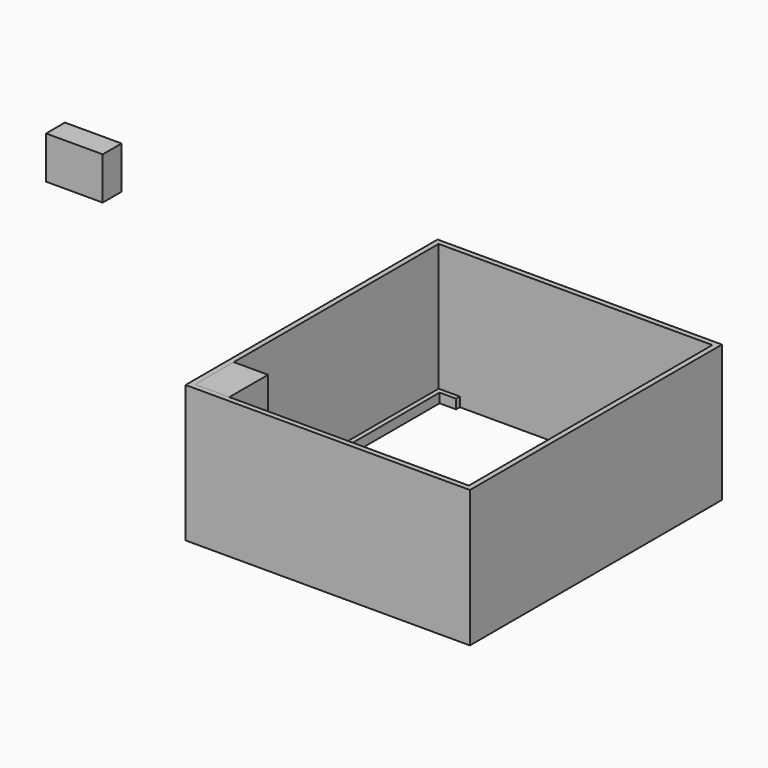
from build123d import *

# Parameters (mm, degrees)
F2_DEPTH     = 203.2
F4_W         = 6121.4
F4_H         = 6781.8
F4_W_2       = 5892.8
F4_H_2       = 6553.2
F5_DEPTH     = 2946.4
F6_W         = 736.6
F6_H         = 1041.4
F7_DEPTH     = 2946.4
F8_W         = 1219.2
F8_H         = 508
F8_W_2       = 28.8176558291
F8_H_2       = 190.1743183326
F8_TEXT_SIZE = 355.362229877
F9_DEPTH     = 914.4


# Not quite as in the source:
# - Text() gives the source's letters only with a copy of the font that has no kerning and outlines rounded to 1/6400 em; it was checked with that copy


with BuildPart() as f2:
    # F1 (on face) → F2 (new body)
    with BuildSketch(Plane.XY):
        Polygon((2515.7309795082, 3987.9328036621), (2845.9309795082, 3987.9328036621), (2845.9309795082, -2362.0671963379), (-2843.6690204918, -2362.0671963379), (-2843.6690204918, 3987.9328036621), (-2488.0690204918, 3987.9328036621), (-2488.0690204918, 4089.5328036621), (-2945.2690204918, 4089.5328036621), (-2945.2690204918, -2463.6671963379), (2947.5309795082, -2463.6671963379), (2947.5309795082, 4089.5328036621), (2515.7309795082, 4089.5328036621), align=None)
    extrude(amount=F2_DEPTH)

    # F4 (on face) → F5 (join)
    with BuildSketch(Plane.XY):
        with Locations((1.1309795082, 812.9328036621)):
            Rectangle(F4_W, F4_H)
        with Locations((1.1309795082, 812.9328036621)):
            Rectangle(F4_W_2, F4_H_2, mode=Mode.SUBTRACT)
    extrude(amount=F5_DEPTH)


with BuildPart() as f7:
    # F6 (on face) → F7 (new body)
    with BuildSketch(Plane.XY):
        with Locations((-2576.9690204918, -1942.9671963379)):
            Rectangle(F6_W, F6_H)
    extrude(amount=F7_DEPTH)


with BuildPart() as f9:
    # F8 (on face) → F9 (new body)
    with BuildSketch(Plane.XY):
        with Locations((-12440.1019524327, 6409.4748497009)):
            Rectangle(F8_W, F8_H)
        with BuildLine():
            add(Edge.make_bspline(
                [(-12936.3292676086, 6262.9570359261), (-12952.9868721341, 6244.8280096675), (-12984.2476432936, 6244.8280096675)],
                knots=[0, 0, 0, 1, 1, 1], degree=2))
            add(Edge.make_bspline(
                [(-12984.2476432936, 6244.8280096675), (-13000.5165703802, 6244.8280096675), (-13009.9003542629, 6249.4921389346)],
                knots=[0, 0, 0, 1, 1, 1], degree=2))
            Line((-13009.9003542629, 6249.4921389346), (-13009.9003542629, 6274.6451217681))
            add(Edge.make_bspline(
                [(-13009.9003542629, 6274.6451217681), (-12997.573726914, 6271.2025501662), (-12984.2476432936, 6271.2025501662)],
                knots=[0, 0, 0, 1, 1, 1], degree=2))
            add(Edge.make_bspline(
                [(-12984.2476432936, 6271.2025501662), (-12967.0347852839, 6271.2025501662), (-12958.0952041886, 6281.6135529946)],
                knots=[0, 0, 0, 1, 1, 1], degree=2))
            add(Edge.make_bspline(
                [(-12958.0952041886, 6281.6135529946), (-12949.1556230932, 6292.024555823), (-12949.1556230932, 6311.6250038147)],
                knots=[0, 0, 0, 1, 1, 1], degree=2))
            Line((-12949.1556230932, 6311.6250038147), (-12949.1556230932, 6565.3203207379))
            Line((-12949.1556230932, 6565.3203207379), (-12919.6716630831, 6565.3203207379))
            Line((-12919.6716630831, 6565.3203207379), (-12919.6716630831, 6314.0681191451))
            add(Edge.make_bspline(
                [(-12919.6716630831, 6314.0681191451), (-12919.6716630831, 6281.0860621846), (-12936.3292676086, 6262.9570359261)],
                knots=[0, 0, 0, 1, 1, 1], degree=2))
        make_face(mode=Mode.SUBTRACT)
        with BuildLine():
            add(Edge.make_bspline(
                [(-12716.0879731075, 6478.7285398795), (-12692.5729880523, 6452.1596606614), (-12692.5729880523, 6406.9065017005)],
                knots=[0, 0, 0, 1, 1, 1], degree=2))
            add(Edge.make_bspline(
                [(-12692.5729880523, 6406.9065017005), (-12692.5729880523, 6360.376259726), (-12715.9769224106, 6334.2515832952)],
                knots=[0, 0, 0, 1, 1, 1], degree=2))
            add(Edge.make_bspline(
                [(-12715.9769224106, 6334.2515832952), (-12739.380856769, 6308.1269068643), (-12780.6917159922, 6308.1269068643)],
                knots=[0, 0, 0, 1, 1, 1], degree=2))
            add(Edge.make_bspline(
                [(-12780.6917159922, 6308.1269068643), (-12806.2333762646, 6308.1269068643), (-12826.0004003015, 6320.1203821227)],
                knots=[0, 0, 0, 1, 1, 1], degree=2))
            add(Edge.make_bspline(
                [(-12826.0004003015, 6320.1203821227), (-12845.7674243384, 6332.113857381), (-12856.5393419315, 6354.4905727936)],
                knots=[0, 0, 0, 1, 1, 1], degree=2))
            add(Edge.make_bspline(
                [(-12856.5393419315, 6354.4905727936), (-12867.3112595247, 6376.8672882062), (-12867.3112595247, 6406.9065017005)],
                knots=[0, 0, 0, 1, 1, 1], degree=2))
            add(Edge.make_bspline(
                [(-12867.3112595247, 6406.9065017005), (-12867.3112595247, 6453.3812183266), (-12844.0461385374, 6479.3393187121)],
                knots=[0, 0, 0, 1, 1, 1], degree=2))
            add(Edge.make_bspline(
                [(-12844.0461385374, 6479.3393187121), (-12820.7810175502, 6505.2974190977), (-12779.470158327, 6505.2974190977)],
                knots=[0, 0, 0, 1, 1, 1], degree=2))
            add(Edge.make_bspline(
                [(-12779.470158327, 6505.2974190977), (-12739.6029581626, 6505.2974190977), (-12716.0879731075, 6478.7285398795)],
                knots=[0, 0, 0, 1, 1, 1], degree=2))
        make_face(mode=Mode.SUBTRACT)
        with Locations((-12627.6360930771, 6406.712162981)):
            Rectangle(F8_W_2, F8_H_2, mode=Mode.SUBTRACT)
        with BuildLine():
            add(Edge.make_bspline(
                [(-12639.6295683355, 6538.8347295423), (-12644.4880363221, 6543.6099095063), (-12644.4880363221, 6553.3268454795)],
                knots=[0, 0, 0, 1, 1, 1], degree=2))
            add(Edge.make_bspline(
                [(-12644.4880363221, 6553.3268454795), (-12644.4880363221, 6563.210357498), (-12639.6295683355, 6567.8189614167)],
                knots=[0, 0, 0, 1, 1, 1], degree=2))
            add(Edge.make_bspline(
                [(-12639.6295683355, 6567.8189614167), (-12634.7711003489, 6572.4275653354), (-12627.4417543577, 6572.4275653354)],
                knots=[0, 0, 0, 1, 1, 1], degree=2))
            add(Edge.make_bspline(
                [(-12627.4417543577, 6572.4275653354), (-12620.5010858054, 6572.4275653354), (-12615.4760417735, 6567.7356733941)],
                knots=[0, 0, 0, 1, 1, 1], degree=2))
            add(Edge.make_bspline(
                [(-12615.4760417735, 6567.7356733941), (-12610.4509977417, 6563.0437814527), (-12610.4509977417, 6553.3268454795)],
                knots=[0, 0, 0, 1, 1, 1], degree=2))
            add(Edge.make_bspline(
                [(-12610.4509977417, 6553.3268454795), (-12610.4509977417, 6543.6099095063), (-12615.4760417735, 6538.8347295423)],
                knots=[0, 0, 0, 1, 1, 1], degree=2))
            add(Edge.make_bspline(
                [(-12615.4760417735, 6538.8347295423), (-12620.5010858054, 6534.0595495784), (-12627.4417543577, 6534.0595495784)],
                knots=[0, 0, 0, 1, 1, 1], degree=2))
            add(Edge.make_bspline(
                [(-12627.4417543577, 6534.0595495784), (-12634.7711003489, 6534.0595495784), (-12639.6295683355, 6538.8347295423)],
                knots=[0, 0, 0, 1, 1, 1], degree=2))
        make_face(mode=Mode.SUBTRACT)
        with BuildLine():
            Line((-12393.1803093809, 6311.6250038147), (-12421.99796521, 6311.6250038147))
            Line((-12421.99796521, 6311.6250038147), (-12421.99796521, 6434.6691759096))
            add(Edge.make_bspline(
                [(-12421.99796521, 6434.6691759096), (-12421.99796521, 6457.8787715485), (-12432.5755440837, 6469.3447559968)],
                knots=[0, 0, 0, 1, 1, 1], degree=2))
            add(Edge.make_bspline(
                [(-12432.5755440837, 6469.3447559968), (-12443.1531229574, 6480.8107404452), (-12465.7519397636, 6480.8107404452)],
                knots=[0, 0, 0, 1, 1, 1], degree=2))
            add(Edge.make_bspline(
                [(-12465.7519397636, 6480.8107404452), (-12495.5690518642, 6480.8107404452), (-12509.4503889688, 6464.6806267297)],
                knots=[0, 0, 0, 1, 1, 1], degree=2))
            add(Edge.make_bspline(
                [(-12509.4503889688, 6464.6806267297), (-12523.3317260734, 6448.5505130142), (-12523.3317260734, 6411.4040549224)],
                knots=[0, 0, 0, 1, 1, 1], degree=2))
            Line((-12523.3317260734, 6411.4040549224), (-12523.3317260734, 6311.6250038147))
            Line((-12523.3317260734, 6311.6250038147), (-12552.1493819025, 6311.6250038147))
            Line((-12552.1493819025, 6311.6250038147), (-12552.1493819025, 6501.7993221473))
            Line((-12552.1493819025, 6501.7993221473), (-12528.71768487, 6501.7993221473))
            Line((-12528.71768487, 6501.7993221473), (-12524.0535556028, 6475.7579337392))
            Line((-12524.0535556028, 6475.7579337392), (-12522.6654218924, 6475.7579337392))
            add(Edge.make_bspline(
                [(-12522.6654218924, 6475.7579337392), (-12513.7813661454, 6489.805846889), (-12497.8178284752, 6497.5516329933)],
                knots=[0, 0, 0, 1, 1, 1], degree=2))
            add(Edge.make_bspline(
                [(-12497.8178284752, 6497.5516329933), (-12481.8542908049, 6505.2974190977), (-12462.2538428133, 6505.2974190977)],
                knots=[0, 0, 0, 1, 1, 1], degree=2))
            add(Edge.make_bspline(
                [(-12462.2538428133, 6505.2974190977), (-12427.8836521424, 6505.2974190977), (-12410.5319807616, 6488.7231025948)],
                knots=[0, 0, 0, 1, 1, 1], degree=2))
            add(Edge.make_bspline(
                [(-12410.5319807616, 6488.7231025948), (-12393.1803093809, 6472.148786092), (-12393.1803093809, 6435.6686321812)],
                knots=[0, 0, 0, 1, 1, 1], degree=2))
            Line((-12393.1803093809, 6435.6686321812), (-12393.1803093809, 6311.6250038147))
        make_face(mode=Mode.SUBTRACT)
        with BuildLine():
            add(Edge.make_bspline(
                [(-12295.0114933774, 6341.136726499), (-12286.8492671599, 6331.9472813358), (-12272.6347779648, 6331.9472813358)],
                knots=[0, 0, 0, 1, 1, 1], degree=2))
            add(Edge.make_bspline(
                [(-12272.6347779648, 6331.9472813358), (-12264.9722798831, 6331.9472813358), (-12257.8650352856, 6333.0577883042)],
                knots=[0, 0, 0, 1, 1, 1], degree=2))
            add(Edge.make_bspline(
                [(-12257.8650352856, 6333.0577883042), (-12250.757790688, 6334.1682952725), (-12246.5933895566, 6335.3898529377)],
                knots=[0, 0, 0, 1, 1, 1], degree=2))
            Line((-12246.5933895566, 6335.3898529377), (-12246.5933895566, 6313.3462896157))
            add(Edge.make_bspline(
                [(-12246.5933895566, 6313.3462896157), (-12251.2575188238, 6311.1252756789), (-12260.3636759644, 6309.6260912716)],
                knots=[0, 0, 0, 1, 1, 1], degree=2))
            add(Edge.make_bspline(
                [(-12260.3636759644, 6309.6260912716), (-12269.469833105, 6308.1269068643), (-12276.7991790962, 6308.1269068643)],
                knots=[0, 0, 0, 1, 1, 1], degree=2))
            add(Edge.make_bspline(
                [(-12276.7991790962, 6308.1269068643), (-12331.9358500755, 6308.1269068643), (-12331.9358500755, 6366.2619466583)],
                knots=[0, 0, 0, 1, 1, 1], degree=2))
            Line((-12331.9358500755, 6366.2619466583), (-12331.9358500755, 6479.4226067348))
            Line((-12331.9358500755, 6479.4226067348), (-12359.1987961489, 6479.4226067348))
            Line((-12359.1987961489, 6479.4226067348), (-12359.1987961489, 6493.3039438393))
            Line((-12359.1987961489, 6493.3039438393), (-12331.9358500755, 6505.2974190977))
            Line((-12331.9358500755, 6505.2974190977), (-12319.8313241204, 6545.8864487915))
            Line((-12319.8313241204, 6545.8864487915), (-12303.1737195949, 6545.8864487915))
            Line((-12303.1737195949, 6545.8864487915), (-12303.1737195949, 6501.7993221473))
            Line((-12303.1737195949, 6501.7993221473), (-12247.9815232671, 6501.7993221473))
            Line((-12247.9815232671, 6501.7993221473), (-12247.9815232671, 6479.4226067348))
            Line((-12247.9815232671, 6479.4226067348), (-12303.1737195949, 6479.4226067348))
            Line((-12303.1737195949, 6479.4226067348), (-12303.1737195949, 6367.4835043235))
            add(Edge.make_bspline(
                [(-12303.1737195949, 6367.4835043235), (-12303.1737195949, 6350.3261716622), (-12295.0114933774, 6341.136726499)],
                knots=[0, 0, 0, 1, 1, 1], degree=2))
        make_face(mode=Mode.SUBTRACT)
        with BuildLine():
            add(Edge.make_bspline(
                [(-12095.3978658136, 6311.0142249821), (-12109.0015761761, 6308.1269068643), (-12128.2688720773, 6308.1269068643)],
                knots=[0, 0, 0, 1, 1, 1], degree=2))
            add(Edge.make_bspline(
                [(-12128.2688720773, 6308.1269068643), (-12170.4126115267, 6308.1269068643), (-12194.8160021566, 6333.835143182)],
                knots=[0, 0, 0, 1, 1, 1], degree=2))
            add(Edge.make_bspline(
                [(-12194.8160021566, 6333.835143182), (-12219.2193927864, 6359.5433794997), (-12219.2193927864, 6405.1296905511)],
                knots=[0, 0, 0, 1, 1, 1], degree=2))
            add(Edge.make_bspline(
                [(-12219.2193927864, 6405.1296905511), (-12219.2193927864, 6451.1602043899), (-12196.5650506318, 6478.2288117438)],
                knots=[0, 0, 0, 1, 1, 1], degree=2))
            add(Edge.make_bspline(
                [(-12196.5650506318, 6478.2288117438), (-12173.9107084771, 6505.2974190977), (-12135.7092687653, 6505.2974190977)],
                knots=[0, 0, 0, 1, 1, 1], degree=2))
            add(Edge.make_bspline(
                [(-12135.7092687653, 6505.2974190977), (-12100.0064697324, 6505.2974190977), (-12079.1844640755, 6481.7824340425)],
                knots=[0, 0, 0, 1, 1, 1], degree=2))
            add(Edge.make_bspline(
                [(-12079.1844640755, 6481.7824340425), (-12058.3624584186, 6458.2674489874), (-12058.3624584186, 6419.7328571851)],
                knots=[0, 0, 0, 1, 1, 1], degree=2))
            Line((-12058.3624584186, 6419.7328571851), (-12058.3624584186, 6401.5205429039))
            Line((-12058.3624584186, 6401.5205429039), (-12189.3467553374, 6401.5205429039))
            add(Edge.make_bspline(
                [(-12189.3467553374, 6401.5205429039), (-12188.4583497627, 6368.0387578077), (-12172.4115240698, 6350.687086427)],
                knots=[0, 0, 0, 1, 1, 1], degree=2))
            add(Edge.make_bspline(
                [(-12172.4115240698, 6350.687086427), (-12156.3646983769, 6333.3354150462), (-12127.2138904573, 6333.3354150462)],
                knots=[0, 0, 0, 1, 1, 1], degree=2))
            add(Edge.make_bspline(
                [(-12127.2138904573, 6333.3354150462), (-12096.508372782, 6333.3354150462), (-12066.5246846361, 6346.1617705309)],
                knots=[0, 0, 0, 1, 1, 1], degree=2))
            Line((-12066.5246846361, 6346.1617705309), (-12066.5246846361, 6320.4535342132))
            add(Edge.make_bspline(
                [(-12066.5246846361, 6320.4535342132), (-12081.7941554512, 6313.9015430998), (-12095.3978658136, 6311.0142249821)],
                knots=[0, 0, 0, 1, 1, 1], degree=2))
        make_face(mode=Mode.SUBTRACT)
        with BuildLine():
            add(Edge.make_bspline(
                [(-11955.2518864059, 6495.2195683598), (-11940.3155676814, 6505.2974190977), (-11922.4364054907, 6505.2974190977)],
                knots=[0, 0, 0, 1, 1, 1], degree=2))
            add(Edge.make_bspline(
                [(-11922.4364054907, 6505.2974190977), (-11909.7766260513, 6505.2974190977), (-11899.7265379876, 6503.1874558578)],
                knots=[0, 0, 0, 1, 1, 1], degree=2))
            Line((-11899.7265379876, 6503.1874558578), (-11903.7243630737, 6476.4797632686))
            add(Edge.make_bspline(
                [(-11903.7243630737, 6476.4797632686), (-11915.4957369384, 6479.0894546443), (-11924.5463687306, 6479.0894546443)],
                knots=[0, 0, 0, 1, 1, 1], degree=2))
            add(Edge.make_bspline(
                [(-11924.5463687306, 6479.0894546443), (-11947.6449136726, 6479.0894546443), (-11964.024891456, 6460.3496495531)],
                knots=[0, 0, 0, 1, 1, 1], degree=2))
            add(Edge.make_bspline(
                [(-11964.024891456, 6460.3496495531), (-11980.4048692394, 6441.6098444619), (-11980.4048692394, 6413.6805942075)],
                knots=[0, 0, 0, 1, 1, 1], degree=2))
            Line((-11980.4048692394, 6413.6805942075), (-11980.4048692394, 6311.6250038147))
            Line((-11980.4048692394, 6311.6250038147), (-12009.2225250685, 6311.6250038147))
            Line((-12009.2225250685, 6311.6250038147), (-12009.2225250685, 6501.7993221473))
            Line((-12009.2225250685, 6501.7993221473), (-11985.4576759454, 6501.7993221473))
            Line((-11985.4576759454, 6501.7993221473), (-11982.1261550403, 6466.5962512501))
            Line((-11982.1261550403, 6466.5962512501), (-11980.7380213299, 6466.5962512501))
            add(Edge.make_bspline(
                [(-11980.7380213299, 6466.5962512501), (-11970.1882051304, 6485.1417176218), (-11955.2518864059, 6495.2195683598)],
                knots=[0, 0, 0, 1, 1, 1], degree=2))
        make_face(mode=Mode.SUBTRACT)
        with BuildLine():
            add(Edge.make_bspline(
                [(-12823.0297941611, 6462.2375113993), (-12837.4386220756, 6443.6642823534), (-12837.4386220756, 6406.9065017005)],
                knots=[0, 0, 0, 1, 1, 1], degree=2))
            add(Edge.make_bspline(
                [(-12837.4386220756, 6406.9065017005), (-12837.4386220756, 6370.4263477897), (-12822.8632181159, 6351.353390608)],
                knots=[0, 0, 0, 1, 1, 1], degree=2))
            add(Edge.make_bspline(
                [(-12822.8632181159, 6351.353390608), (-12808.287814156, 6332.2804334263), (-12780.0254118111, 6332.2804334263)],
                knots=[0, 0, 0, 1, 1, 1], degree=2))
            add(Edge.make_bspline(
                [(-12780.0254118111, 6332.2804334263), (-12751.7074841178, 6332.2804334263), (-12737.0487921354, 6351.2701025854)],
                knots=[0, 0, 0, 1, 1, 1], degree=2))
            add(Edge.make_bspline(
                [(-12737.0487921354, 6351.2701025854), (-12722.390100153, 6370.2597717444), (-12722.390100153, 6406.9065017005)],
                knots=[0, 0, 0, 1, 1, 1], degree=2))
            add(Edge.make_bspline(
                [(-12722.390100153, 6406.9065017005), (-12722.390100153, 6443.1645542176), (-12737.0487921354, 6461.9876473314)],
                knots=[0, 0, 0, 1, 1, 1], degree=2))
            add(Edge.make_bspline(
                [(-12737.0487921354, 6461.9876473314), (-12751.7074841178, 6480.8107404452), (-12780.3585639016, 6480.8107404452)],
                knots=[0, 0, 0, 1, 1, 1], degree=2))
            add(Edge.make_bspline(
                [(-12780.3585639016, 6480.8107404452), (-12808.6209662466, 6480.8107404452), (-12823.0297941611, 6462.2375113993)],
                knots=[0, 0, 0, 1, 1, 1], degree=2))
        make_face()
        with BuildLine():
            add(Edge.make_bspline(
                [(-12101.3668407686, 6466.6517765986), (-12113.499129398, 6481.1438925357), (-12136.0979462042, 6481.1438925357)],
                knots=[0, 0, 0, 1, 1, 1], degree=2))
            add(Edge.make_bspline(
                [(-12136.0979462042, 6481.1438925357), (-12158.9743897526, 6481.1438925357), (-12172.6058627893, 6466.2353364854)],
                knots=[0, 0, 0, 1, 1, 1], degree=2))
            add(Edge.make_bspline(
                [(-12172.6058627893, 6466.2353364854), (-12186.237335826, 6451.3267804351), (-12188.6804511564, 6424.9522399364)],
                knots=[0, 0, 0, 1, 1, 1], degree=2))
            Line((-12188.6804511564, 6424.9522399364), (-12089.2345521392, 6424.9522399364))
            add(Edge.make_bspline(
                [(-12089.2345521392, 6424.9522399364), (-12089.2345521392, 6452.1596606614), (-12101.3668407686, 6466.6517765986)],
                knots=[0, 0, 0, 1, 1, 1], degree=2))
        make_face()
        with Locations((-12982.1376800537, 6311.6250038147)):
            Text('Jointer', F8_TEXT_SIZE, font='Open Sans', text_align=(TextAlign.LEFT, TextAlign.BOTTOM))
    extrude(amount=F9_DEPTH)


solid = Compound([f2.part, f7.part, f9.part])
